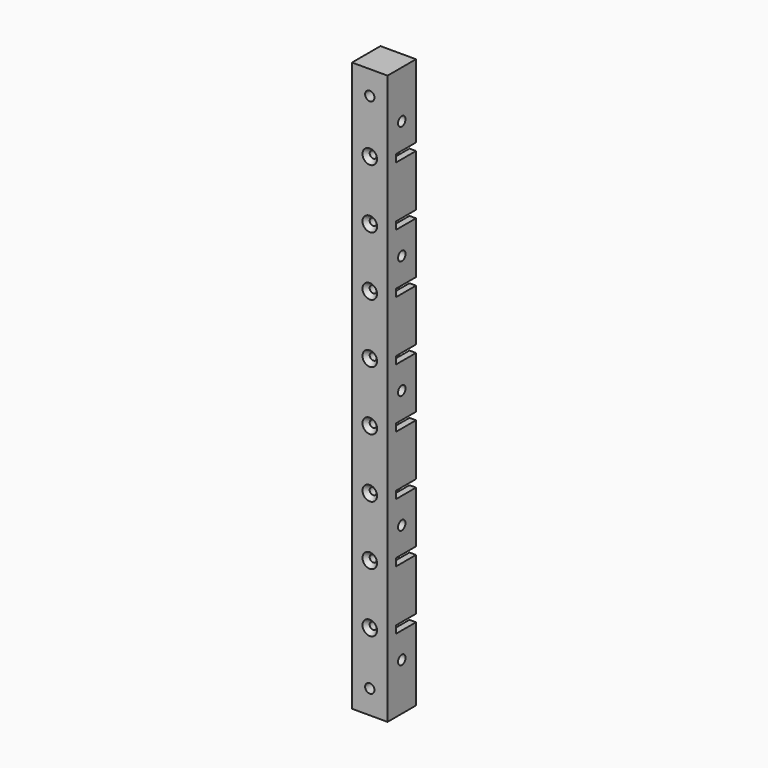
from build123d import *

# Parameters (mm, degrees)
F0_W           = 19.05
F0_H           = 304.8
F1_DEPTH       = 19.05
F3_D           = 5
F5_D           = 3.7973
F5_DEPTH       = 12.7
F5_CSINK_D     = 7.7978
F5_CSINK_ANGLE = 82
F5_TIP         = 1.1408240143
F6_W           = 31.75
F6_H           = 317.5
F6_W_2         = 23.05
F6_H_2         = 308.8
F6_W_3         = 13.335
F6_H_3         = 4
F6_W_4         = 0.9525
F7_DEPTH       = 6.35
F4_R           = 6.35
F8_DEPTH       = 12.7
F10_D          = 5


with BuildPart() as f1:
    # F0 (on Front) → F1 (new body)
    with BuildSketch(Plane.XZ):
        Rectangle(F0_W, F0_H)
    extrude(amount=-F1_DEPTH)

    # F3 (through all)
    with Locations(Plane.YZ.offset(9.525)):
        with Locations((9.525, 127), (9.525, 63.5), (9.525, 0), (9.525, -63.5), (9.525, -127)):
            Hole(F3_D / 2)

    # F5
    with Locations(Plane.XZ):
        with Locations((0, 111.125), (0, 79.375), (0, 47.625), (0, 15.875), (0, -15.875), (0, -47.625), (0, -79.375), (0, -111.125)):
            CounterSinkHole(F5_D / 2, F5_CSINK_D / 2, depth=F5_DEPTH, counter_sink_angle=F5_CSINK_ANGLE)
            with Locations((0, 0, -(F5_DEPTH + F5_TIP / 2))):  # 118° drill point
                Cone(0, F5_D / 2, F5_TIP, mode=Mode.SUBTRACT)

    # F6 (on face) → F7 (cut)
    with BuildSketch(Plane.YZ.offset(9.525)):
        with Locations((9.525, 0)):
            Rectangle(F6_W, F6_H)
        with Locations((9.525, 0)):
            Rectangle(F6_W_2, F6_H_2, mode=Mode.SUBTRACT)
        with Locations((9.525, 0)):
            Rectangle(F6_W_2, F6_H_2)
        Polygon((20.0025, 13.875), (19.05, 13.875), (19.05, -13.875), (20.0025, -13.875), (20.0025, -17.875), (19.05, -17.875), (19.05, -45.625), (20.0025, -45.625), (20.0025, -49.625), (19.05, -49.625), (19.05, -77.375), (20.0025, -77.375), (20.0025, -81.375), (19.05, -81.375), (19.05, -109.125), (20.0025, -109.125), (20.0025, -113.125), (19.05, -113.125), (19.05, -152.4), (0, -152.4), (0, 152.4), (19.05, 152.4), (19.05, 113.125), (20.0025, 113.125), (20.0025, 109.125), (19.05, 109.125), (19.05, 81.375), (20.0025, 81.375), (20.0025, 77.375), (19.05, 77.375), (19.05, 49.625), (20.0025, 49.625), (20.0025, 45.625), (19.05, 45.625), (19.05, 17.875), (20.0025, 17.875), align=None, mode=Mode.SUBTRACT)
        with Locations((12.3825, -15.875)):
            Rectangle(F6_W_3, F6_H_3)
        with Locations((12.3825, 47.625)):
            Rectangle(F6_W_3, F6_H_3)
        with Locations((12.3825, -47.625)):
            Rectangle(F6_W_3, F6_H_3)
        Polygon((5.715, 77.375), (19.05, 77.375), (19.05, 77.3812195068), (19.05, 81.375), (5.715, 81.375), align=None)
        with Locations((12.3825, -79.375)):
            Rectangle(F6_W_3, F6_H_3)
        with Locations((12.3825, -111.125)):
            Rectangle(F6_W_3, F6_H_3)
        with Locations((12.3825, 111.125)):
            Rectangle(F6_W_3, F6_H_3)
        Polygon((5.715, 17.875), (5.715, 13.8770895111), (19.05, 13.8751393007), (19.05, 17.875), align=None)
        with Locations((19.52625, 47.625)):
            Rectangle(F6_W_4, F6_H_3)
        with Locations((19.52625, 111.125)):
            Rectangle(F6_W_4, F6_H_3)
        Polygon((19.05, 17.875), (19.05, 13.8751393007), (20.0025, 13.875), (20.0025, 17.875), align=None)
        Polygon((19.05, 77.3812195068), (20.0025, 77.375), (20.0025, 81.375), (19.05, 81.375), align=None)
    extrude(amount=-F7_DEPTH, mode=Mode.SUBTRACT)

    # F4 (on face) → F8 (cut)
    with BuildSketch(Plane(origin=(0, 19.05, 0), x_dir=(-1, 0, 0), z_dir=(0, 1, 0))):
        with Locations((0, 111.125)):
            Circle(F4_R)
        with Locations((0, 79.375)):
            Circle(F4_R)
        with Locations((0, 47.625)):
            Circle(F4_R)
        with Locations((0, 15.875)):
            Circle(F4_R)
        with Locations((0, -47.625)):
            Circle(F4_R)
        with Locations((0, -79.375)):
            Circle(F4_R)
        with Locations((0, -111.125)):
            Circle(F4_R)
        with Locations((0, -15.875)):
            Circle(F4_R)
    extrude(amount=-F8_DEPTH, mode=Mode.SUBTRACT)

    # F10 (through all)
    with Locations(Plane(origin=(0, 19.05, 0), x_dir=(-1, 0, 0), z_dir=(0, 1, 0))):
        with Locations((0, 139.7), (0, -139.7)):
            Hole(F10_D / 2)


solid = f1.part
